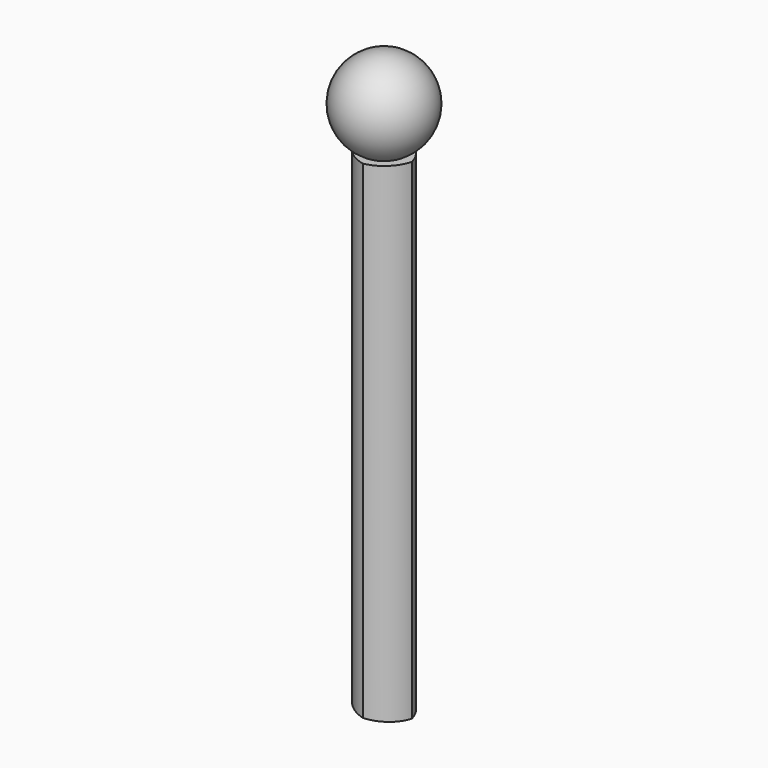
from build123d import *

# Parameters (mm, degrees)
F3_DEPTH      = 3.81
F3_DEPTH_BACK = 3.81
F4_T4_DEPTH   = 81.9290237066
F4_T9_DEPTH   = 81.9290237066
F4_T14_DEPTH  = 81.28
F4_T19_DEPTH  = 81.28


# Not quite as in the source:
# - a fillet or chamfer that OpenCascade refuses, or shapes differently, is made with other operations: its cross-section is extruded or revolved along the edge and cut away or added


with BuildPart() as f1:
    # F0 (on Front) → F1 (revolve)
    with BuildSketch(Plane.XZ):
        with BuildLine():
            Line((0, -6.35), (0, 6.35))
            ThreePointArc((0, 6.35), (-6.35, 0), (0, -6.35))
        make_face()
    revolve(axis=Axis((0, 0, 0), (0, 0, -1)))

    # F2 (on Front) → F3 (join, two sides)
    with BuildSketch(Plane.XZ) as f3_sk:
        Polygon((4.1104733182, -5.9445748625), (-4.1104737839, -5.9445748625), (-4.1104737839, -74.5245748625), (4.1104733182, -75.1735985691), align=None)
    extrude(amount=-F3_DEPTH)
    extrude(f3_sk.sketch, amount=F3_DEPTH_BACK)

    # F4: fillet of radius 5.08 on 4 edges, made by hand


with BuildPart() as f4_tool2:
    # F4_s3 → F4_t4 (new body)
    with BuildSketch(Plane.XY.offset(-87.8735985691)):
        with BuildLine():
            ThreePointArc((4.1104733182, 1.27), (2.6225757666, -2.3221024484), (-0.9695266818, -3.81))
            Line((-0.9695266818, -3.81), (-0.9695266818, -3.9116))
            Line((-0.9695266818, -3.9116), (4.2120733182, -3.9116))
            Line((4.2120733182, -3.9116), (4.2120733182, 1.27))
            Line((4.2120733182, 1.27), (4.1104733182, 1.27))
        make_face()
    extrude(amount=F4_T4_DEPTH)

    split(bisect_by=Plane(origin=(-5.8725507458, 0, -74.3854631875), x_dir=(0, 1, 0), z_dir=(0.0787026743, 0, 0.9968981337)), keep=Keep.TOP)


with BuildPart() as f1_1:
    add(f1.part)

    # F4_t1: cut F4_tool2
    add(f4_tool2.part, mode=Mode.SUBTRACT)


with BuildPart() as f4_tool7:
    # F4_s8 → F4_t9 (new body)
    with BuildSketch(Plane.XY.offset(-87.8735985691)):
        with BuildLine():
            ThreePointArc((4.1104733182, -1.27), (2.6225757666, 2.3221024484), (-0.9695266818, 3.81))
            Line((-0.9695266818, 3.81), (-0.9695266818, 3.9116))
            Line((-0.9695266818, 3.9116), (4.2120733182, 3.9116))
            Line((4.2120733182, 3.9116), (4.2120733182, -1.27))
            Line((4.2120733182, -1.27), (4.1104733182, -1.27))
        make_face()
    extrude(amount=F4_T9_DEPTH)

    split(bisect_by=Plane(origin=(-5.8725507458, 0, -74.3854631875), x_dir=(0, 1, 0), z_dir=(0.0787026743, 0, 0.9968981337)), keep=Keep.TOP)


with BuildPart() as f1_2:
    add(f1_1.part)

    # F4_t6: cut F4_tool7
    add(f4_tool7.part, mode=Mode.SUBTRACT)


with BuildPart() as f4_tool12:
    # F4_s13 → F4_t14 (new body)
    with BuildSketch(Plane.XY.offset(-5.9445748625)):
        with BuildLine():
            ThreePointArc((0.9695262161, -3.81), (-2.6225762323, -2.3221024484), (-4.1104737839, 1.27))
            Line((-4.1104737839, 1.27), (-4.2120737839, 1.27))
            Line((-4.2120737839, 1.27), (-4.2120737839, -3.9116))
            Line((-4.2120737839, -3.9116), (0.9695262161, -3.9116))
            Line((0.9695262161, -3.9116), (0.9695262161, -3.81))
        make_face()
    extrude(amount=-F4_T14_DEPTH)

    split(bisect_by=Plane(origin=(-5.8725507458, 0, -74.3854631875), x_dir=(0, 1, 0), z_dir=(0.0787026743, 0, 0.9968981337)), keep=Keep.TOP)


with BuildPart() as f1_3:
    add(f1_2.part)

    # F4_t11: cut F4_tool12
    add(f4_tool12.part, mode=Mode.SUBTRACT)


with BuildPart() as f4_tool17:
    # F4_s18 → F4_t19 (new body)
    with BuildSketch(Plane.XY.offset(-5.9445748625)):
        with BuildLine():
            ThreePointArc((0.9695262161, 3.81), (-2.6225762323, 2.3221024484), (-4.1104737839, -1.27))
            Line((-4.1104737839, -1.27), (-4.2120737839, -1.27))
            Line((-4.2120737839, -1.27), (-4.2120737839, 3.9116))
            Line((-4.2120737839, 3.9116), (0.9695262161, 3.9116))
            Line((0.9695262161, 3.9116), (0.9695262161, 3.81))
        make_face()
    extrude(amount=-F4_T19_DEPTH)

    split(bisect_by=Plane(origin=(-5.8725507458, 0, -74.3854631875), x_dir=(0, 1, 0), z_dir=(0.0787026743, 0, 0.9968981337)), keep=Keep.TOP)


with BuildPart() as f1_4:
    add(f1_3.part)

    # F4_t16: cut F4_tool17
    add(f4_tool17.part, mode=Mode.SUBTRACT)


solid = f1_4.part
